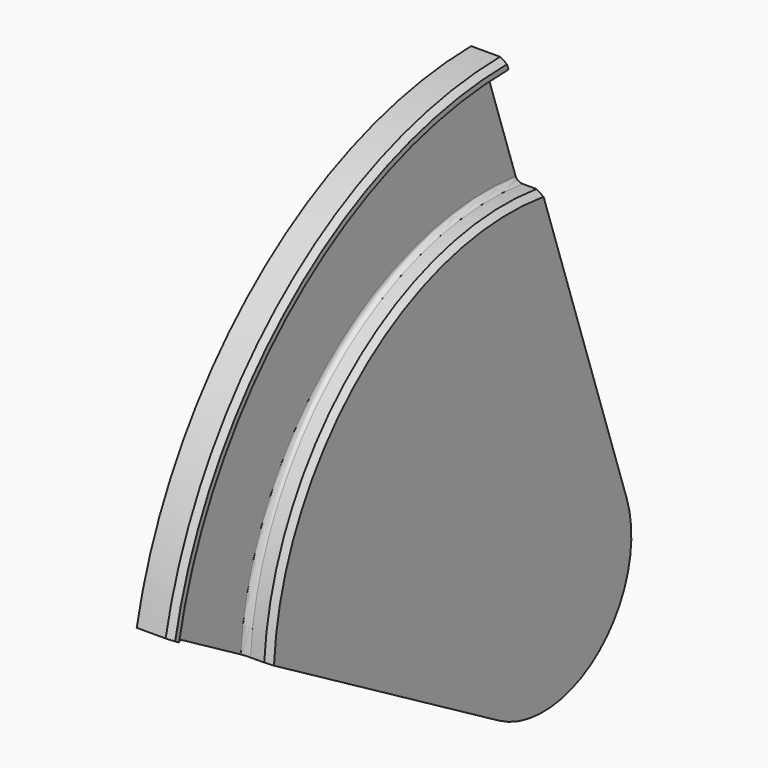
from build123d import *

# Parameters (mm, degrees)
F1_DEPTH     = 2.37
F3_DEPTH     = 2.37
F5_DEPTH     = 2.25
F6_DEPTH     = 0.75
F7_SIZE      = 0.5
F8_T4_ANGLE  = 81.836383008
F8_T10_ANGLE = 99.1168662244
F10_DEPTH    = 3.12


# Not quite as in the source:
# - a fillet or chamfer that OpenCascade refuses, or shapes differently, is made with other operations: its cross-section is extruded or revolved along the edge and cut away or added


with BuildPart() as f1:
    # F0 (on Right) → F1 (new body)
    with BuildSketch(Plane.YZ):
        with BuildLine():
            ThreePointArc((-46.5614527995, 89.8296507657), (-59.272592692, 87.6283434753), (-70.5032497848, 81.2808106933))
            Line((-70.5032497848, 81.2808106933), (-46.5614527995, 52.0296507657))
            Line((-46.5614527995, 52.0296507657), (-42.2863249385, 46.8064651858))
            ThreePointArc((-42.2863249385, 46.8064651858), (-37.3697308445, 54.2738686288), (-37.5751261635, 63.2121472344))
            Line((-37.5751261635, 63.2121472344), (-46.5614527995, 89.8296507657))
        make_face()
        with BuildLine():
            Line((-46.5614527995, 52.0296507657), (-70.5032497848, 81.2808106933))
            ThreePointArc((-70.5032497848, 81.2808106933), (-78.9453750126, 71.5263577209), (-83.6157032002, 59.501098232))
            Line((-83.6157032002, 59.501098232), (-59.2995451707, 45.4309163095))
            ThreePointArc((-59.2995451707, 45.4309163095), (-50.5782061954, 43.4628568222), (-42.2863249385, 46.8064651858))
            Line((-42.2863249385, 46.8064651858), (-46.5614527995, 52.0296507657))
        make_face()
    extrude(amount=F1_DEPTH)

    # F2 (on face) → F3 (join)
    with BuildSketch(Plane(origin=(0, 0, 0), x_dir=(0, -1, 0), z_dir=(-1, 0, 0))):
        with BuildLine():
            ThreePointArc((84.0721339402, 59.7652050675), (70.8199402211, 81.6677307982), (46.7301322311, 90.3292793181))
            Line((46.7301322311, 90.3292793181), (46.5614527995, 89.8296507657))
            ThreePointArc((46.5614527995, 89.8296507657), (70.5032497848, 81.2808106933), (83.6157032002, 59.501098232))
            Line((83.6157032002, 59.501098232), (84.0721339402, 59.7652050675))
        make_face()
        with BuildLine():
            ThreePointArc((84.9830454985, 60.2922904452), (71.4533210937, 82.4415710079), (47.0667704776, 91.3264019551))
            Line((47.0667704776, 91.3264019551), (46.7301322311, 90.3292793181))
            ThreePointArc((46.7301322311, 90.3292793181), (70.8199402211, 81.6677307982), (84.0721339402, 59.7652050675))
            Line((84.0721339402, 59.7652050675), (84.9830454985, 60.2922904452))
        make_face()
    extrude(amount=-F3_DEPTH)

    # F4 (on face) → F5 (cut)
    with BuildSketch(Plane.YZ.offset(2.37)):
        with BuildLine():
            ThreePointArc((-73.802497152, 53.8228330154), (-63.8527506222, 73.1554884912), (-42.9348652938, 79.0876969454))
            Line((-42.9348652938, 79.0876969454), (-46.7301322311, 90.3292793181))
            ThreePointArc((-46.7301322311, 90.3292793181), (-70.8199402211, 81.6677307982), (-84.0721339402, 59.7652050675))
            Line((-84.0721339402, 59.7652050675), (-73.802497152, 53.8228330154))
        make_face()
    extrude(amount=-F5_DEPTH, mode=Mode.SUBTRACT)

    # F6 (add): a face of the model
    f6_faces = [f1.faces().sort_by_distance(p)[0] for p in [
        (0, -58.3598378742, 66.4444605195),
    ]]
    extrude(f6_faces, amount=F6_DEPTH)

    # F7
    f7_edges = [f1.edges().sort_by_distance(p)[0] for p in [
        (2.37, -71.453321, 82.441571),
        (2.37, -63.852751, 73.155488),
    ]]
    chamfer(f7_edges, length=F7_SIZE)

    # F8: fillet of radius 0.5 on 2 edges, made by hand


with BuildPart() as f8_tool2:
    # F8_s3 → F8_t4 (revolve)
    with BuildSketch(Plane(origin=(0, -47.9930028953, 1.3558158365), x_dir=(1, 0, 0), z_dir=(0, 0.9996011995, -0.0282390152))):
        with BuildLine():
            ThreePointArc((0.62, -88.9940517429), (0.2664466094, -88.8476051335), (0.12, -88.4940517429))
            Line((0.12, -88.4940517429), (0.12, -88.9940517429))
            Line((0.12, -88.9940517429), (0.62, -88.9940517429))
        make_face()
    revolve(axis=Axis((0.12, -46.5614527995, 52.0296507657), (1, 0, 0)), revolution_arc=F8_T4_ANGLE)

    split(bisect_by=Plane(origin=(0, 4.8196318055, 8.3293115378), x_dir=(1, 0, 0), z_dir=(0, 0.5008338095, 0.8655434681)), keep=Keep.TOP)

    split(bisect_by=Plane(origin=(0, -14.5730530493, -4.9200036596), x_dir=(1, 0, 0), z_dir=(0, -0.947460791, -0.3198719268)), keep=Keep.TOP)


with BuildPart() as f1_1:
    add(f1.part)

    # F8_t1: union F8_tool2
    add(f8_tool2.part)


with BuildPart() as f8_tool8:
    # F8_s9 → F8_t10 (revolve)
    with BuildSketch(Plane(origin=(0, 1.0178886406, 51.0815497106), x_dir=(1, 0, 0), z_dir=(0, -0.0199227826, -0.9998015217))):
        with BuildLine():
            ThreePointArc((0.12, 75.388786783), (0.2664466094, 75.0352333924), (0.62, 74.888786783))
            Line((0.62, 74.888786783), (0.12, 74.888786783))
            Line((0.12, 74.888786783), (0.12, 75.388786783))
        make_face()
    revolve(axis=Axis((0.12, -46.5614527995, 52.0296507657), (-1, 0, 0)), revolution_arc=F8_T10_ANGLE)

    split(bisect_by=Plane(origin=(0, 4.8196318055, 8.3293115378), x_dir=(1, 0, 0), z_dir=(0, 0.5008338095, 0.8655434681)), keep=Keep.TOP)

    split(bisect_by=Plane(origin=(0, -14.5730530493, -4.9200036596), x_dir=(1, 0, 0), z_dir=(0, -0.947460791, -0.3198719268)), keep=Keep.TOP)


with BuildPart() as f1_2:
    add(f1_1.part)

    # F8_t7: union F8_tool8
    add(f8_tool8.part)

    # F9 (on face) → F10 (join)
    with BuildSketch(Plane(origin=(-0.75, 0, 0), x_dir=(0, -1, 0), z_dir=(-1, 0, 0))):
        with BuildLine():
            ThreePointArc((59.2995451707, 45.4309163095), (42.2863249385, 46.8064651858), (37.5751261635, 63.2121472344))
            Line((37.5751261635, 63.2121472344), (33.3301843859, 50.6386277829))
            ThreePointArc((33.3301843859, 50.6386277829), (36.4709835693, 39.7015064172), (47.8131303907, 38.784473833))
            Line((47.8131303907, 38.784473833), (59.2995451707, 45.4309163095))
        make_face()
    extrude(amount=-F10_DEPTH)


solid = f1_2.part
